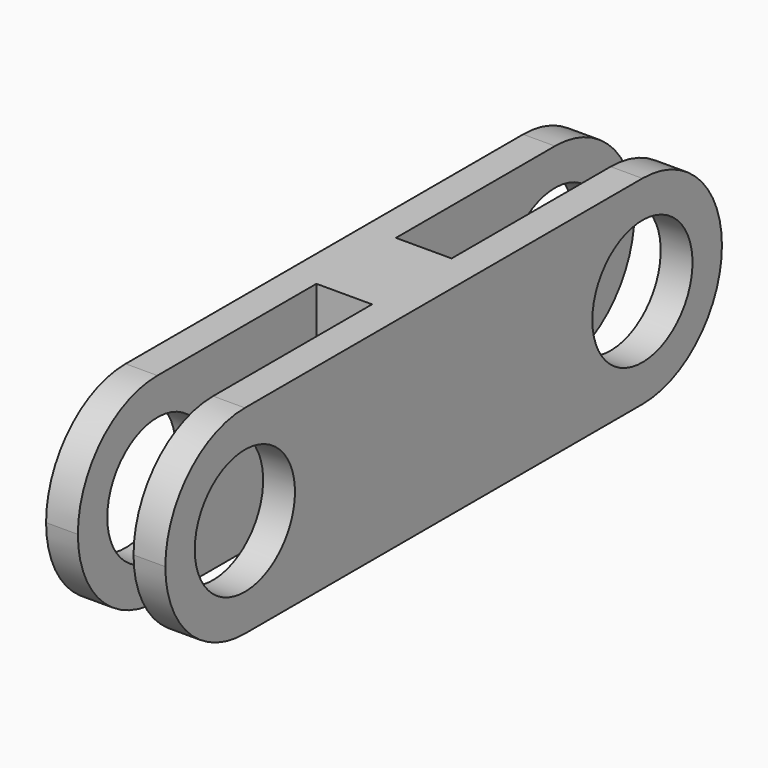
from build123d import *

# Parameters (mm, degrees)
F1_DEPTH   = 0.889
F3_DEPTH   = 6.35
F4_R       = 3.17499
F7_D       = 4
F7_ON_F6_D = 4


# Not quite as in the source:
# - a fillet or chamfer is up to 0.001 mm smaller than in the source, because OpenCascade refuses the exact size
# - a feature names something its author has since deleted; it is built from what else it names


with BuildPart() as f1:
    # F0 (on Right) → F1 (new body, symmetric)
    with BuildSketch(Plane.YZ):
        Polygon((1.5875, 3.175), (-1.5875, 3.175), (-1.5875, 0), (0, 0), (1.5875, 0), align=None)
        Polygon((0, 0), (-1.5875, 0), (-1.5875, -3.175), (1.5875, -3.175), (1.5875, 0), align=None)
    extrude(amount=F1_DEPTH, both=True)

    # F2 (on face) → F3 (join)
    with BuildSketch(Plane(origin=(0, 0, -3.175), x_dir=(1, 0, 0), z_dir=(0, 0, -1))):
        Polygon((0.889, 0), (1.905, 0), (1.905, 11.1125), (0.889, 11.1125), (0.889, 1.5875), (-0.889, 1.5875), (-0.889, 11.1125), (-1.905, 11.1125), (-1.905, 0), (-0.889, 0), (0, 0), align=None)
        Polygon((1.905, -11.1125), (1.905, 0), (0.889, 0), (0, 0), (-0.889, 0), (-1.905, 0), (-1.905, -11.1125), (-0.889, -11.1125), (-0.889, -1.5875), (0.889, -1.5875), (0.889, -11.1125), align=None)
    extrude(amount=-F3_DEPTH)

    # F4 (radius 3.175 in the source; OpenCascade refuses exactly that, so slightly less here)
    f4_edges = [f1.edges().sort_by_distance(p)[0] for p in [
        (1.397, -11.1125, 3.175),
        (-1.397, -11.1125, 3.175),
        (1.397, -11.1125, -3.175),
        (-1.397, -11.1125, -3.175),
        (-1.397, 11.1125, -3.175),
        (1.397, 11.1125, -3.175),
        (1.397, 11.1125, 3.175),
        (-1.397, 11.1125, 3.175),
    ]]
    fillet(f4_edges, radius=F4_R)

    # F7 (through all)
    with Locations(Plane.YZ.offset(1.905)):
        with Locations((-7.9375, 0)):
            Hole(F7_D / 2)

    # F7 on F6 (through all)
    with Locations(Plane.YZ.offset(1.905)):
        with Locations((7.9375, 0)):
            Hole(F7_ON_F6_D / 2)


solid = f1.part
